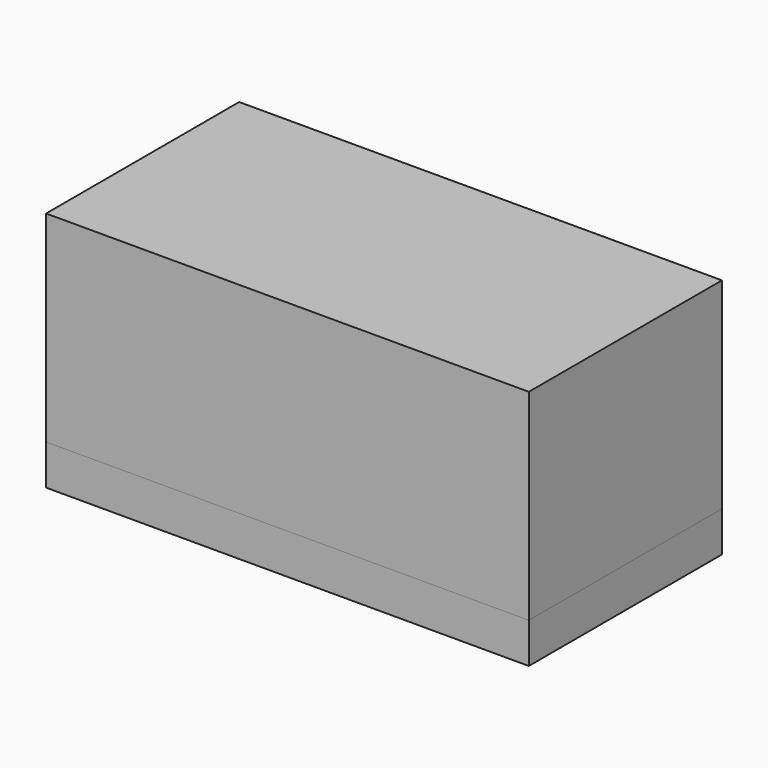
from build123d import *

# Parameters (mm, degrees)
F0_W     = 152.4
F0_H     = 76.2
F1_DEPTH = 76.2
F2_T     = -6.35
F3_W     = 152.4
F3_H     = 76.2
F4_DEPTH = 12.7


# Not quite as in the source:
# - a length typed as a fraction of an inch, garbled in the dataset ("3 / 203.2 mm" for 3/8 in), is restored


with BuildPart() as f1:
    # F0 (on Top) → F1 (new body)
    with BuildSketch(Plane.XY):
        Rectangle(F0_W, F0_H)
    extrude(amount=F1_DEPTH)

    # F2
    f2_openings = [f1.faces().sort_by_distance(p)[0] for p in [
        (0, 0, 0),
    ]]
    offset(amount=F2_T, openings=f2_openings)


with BuildPart() as f4:
    # F3 (on Top) → F4 (new body)
    with BuildSketch(Plane.XY):
        Rectangle(F3_W, F3_H)
    extrude(amount=F4_DEPTH)


solid = Compound([f1.part, f4.part])
